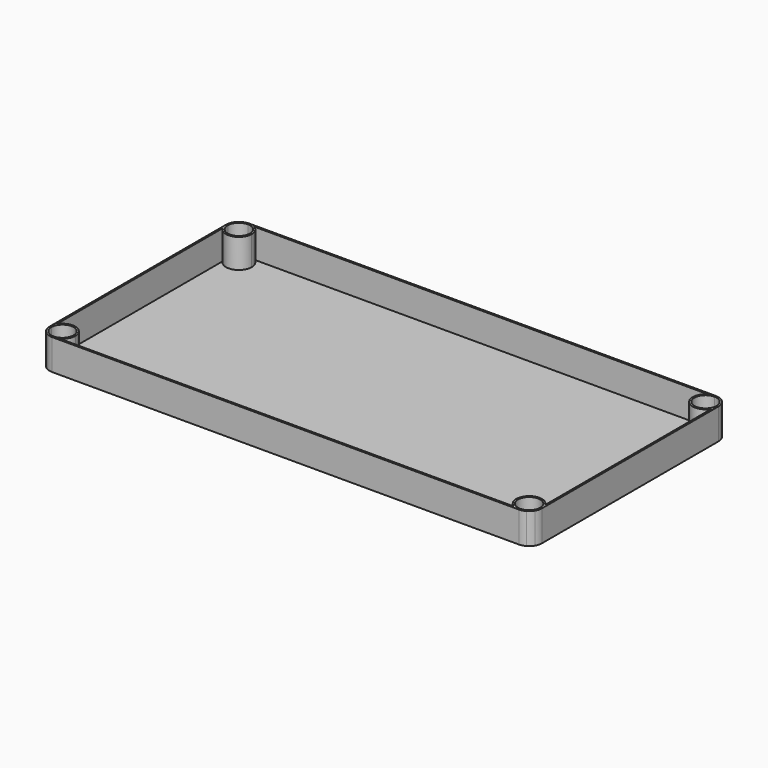
from build123d import *

# Parameters (mm, degrees)
F2_W     = 914.4
F2_H     = 457.2
F3_DEPTH = 57.15
F5_DEPTH = 53.975
F6_DEPTH = 57.15


# Not quite as in the source:
# - a length typed as a fraction of an inch, garbled in the dataset ("3 / 203.2 mm" for 3/8 in), is restored


with BuildPart() as f3:
    # F2 (on Top) → F3 (new body)
    with BuildSketch(Plane.XY):
        with Locations((457.2, 228.6)):
            Rectangle(F2_W, F2_H)
    extrude(amount=F3_DEPTH)

    # F4 (on face) → F5 (cut)
    with BuildSketch(Plane.XY.offset(57.15)):
        with BuildLine():
            ThreePointArc((47.625, 23.8125), (44.4270821412, 11.8930134592), (35.692262203, 3.175))
            Line((35.692262203, 3.175), (878.707737797, 3.175))
            ThreePointArc((878.707737797, 3.175), (873.749519773, 40.650480227), (911.225, 35.692262203))
            Line((911.225, 35.692262203), (911.225, 421.507737797))
            ThreePointArc((911.225, 421.507737797), (873.749519773, 416.549519773), (878.707737797, 454.025))
            Line((878.707737797, 454.025), (35.692262203, 454.025))
            ThreePointArc((35.692262203, 454.025), (44.4270821412, 445.3069865408), (47.625, 433.3875))
            ThreePointArc((47.625, 433.3875), (29.9608610621, 410.3824394154), (3.175, 421.507737797))
            Line((3.175, 421.507737797), (3.175, 35.692262203))
            ThreePointArc((3.175, 35.692262203), (29.9608610621, 46.8175605846), (47.625, 23.8125))
        make_face()
    extrude(amount=-F5_DEPTH, mode=Mode.SUBTRACT)

    # F4 (on face) → F6 (cut)
    with BuildSketch(Plane.XY.offset(57.15)):
        with BuildLine():
            Line((11.932737797, 3.175), (3.175, 3.175))
            Line((3.175, 3.175), (3.175, 11.932737797))
            ThreePointArc((3.175, 11.932737797), (0.8074394304, 17.6641388819), (0, 23.8124998841))
            Line((0, 23.8124998841), (0, 0))
            Line((0, 0), (23.8125, 0))
            ThreePointArc((23.8125, 0), (17.6641389379, 0.8074394154), (11.932737797, 3.175))
        make_face()
        with BuildLine():
            Line((3.175, 11.932737797), (3.175, 3.175))
            Line((3.175, 3.175), (11.932737797, 3.175))
            ThreePointArc((11.932737797, 3.175), (6.974519773, 6.974519773), (3.175, 11.932737797))
        make_face()
        with BuildLine():
            ThreePointArc((3.175, 23.8125001882), (9.2195837367, 9.2195838698), (23.8125, 3.175))
            ThreePointArc((23.8125, 3.175), (38.4054161967, 9.2195838033), (44.45, 23.8125))
            ThreePointArc((44.45, 23.8125), (23.8125000941, 44.45), (3.175, 23.8125001882))
        make_face()
        with BuildLine():
            ThreePointArc((23.8124998376, 454.025), (9.2195837458, 447.9804161393), (3.175, 433.3875))
            ThreePointArc((3.175, 433.3875), (23.8125, 412.75), (44.45, 433.3875))
            ThreePointArc((44.45, 433.3875), (38.4054161393, 447.9804162542), (23.8124998376, 454.025))
        make_face()
        with BuildLine():
            Line((3.175, 454.025), (3.175, 445.267262203))
            ThreePointArc((3.175, 445.267262203), (6.974519773, 450.225480227), (11.932737797, 454.025))
            Line((11.932737797, 454.025), (3.175, 454.025))
        make_face()
        with BuildLine():
            Line((0, 457.2), (0, 433.3875))
            ThreePointArc((0, 433.3875), (0.8074394154, 439.5358610621), (3.175, 445.267262203))
            Line((3.175, 445.267262203), (3.175, 454.025))
            Line((3.175, 454.025), (11.932737797, 454.025))
            ThreePointArc((11.932737797, 454.025), (17.6641390246, 456.3925606078), (23.8125001795, 457.2))
            Line((23.8125001795, 457.2), (0, 457.2))
        make_face()
        with BuildLine():
            ThreePointArc((902.467262203, 454.025), (907.425480227, 450.225480227), (911.225, 445.267262203))
            Line((911.225, 445.267262203), (911.225, 454.025))
            Line((911.225, 454.025), (902.467262203, 454.025))
        make_face()
        with BuildLine():
            ThreePointArc((911.225, 445.267262203), (913.5925605846, 439.5358610621), (914.4, 433.3875))
            Line((914.4, 433.3875), (914.4, 457.2))
            Line((914.4, 457.2), (890.5875, 457.2))
            ThreePointArc((890.5875, 457.2), (896.7358610621, 456.3925605846), (902.467262203, 454.025))
            Line((902.467262203, 454.025), (911.225, 454.025))
            Line((911.225, 454.025), (911.225, 445.267262203))
        make_face()
        with BuildLine():
            ThreePointArc((890.5875, 454.025), (875.9945838033, 418.7945838033), (911.225, 433.3875))
            ThreePointArc((911.225, 433.3875), (905.1804161967, 447.9804161967), (890.5875, 454.025))
        make_face()
        with BuildLine():
            ThreePointArc((911.225, 11.932737797), (907.425480227, 6.974519773), (902.467262203, 3.175))
            Line((902.467262203, 3.175), (911.225, 3.175))
            Line((911.225, 3.175), (911.225, 11.932737797))
        make_face()
        with BuildLine():
            ThreePointArc((902.467262203, 3.175), (896.7358610621, 0.8074394154), (890.5875, 0))
            Line((890.5875, 0), (914.4, 0))
            Line((914.4, 0), (914.4, 23.8125))
            ThreePointArc((914.4, 23.8125), (913.5925605846, 17.6641389379), (911.225, 11.932737797))
            Line((911.225, 11.932737797), (911.225, 3.175))
            Line((911.225, 3.175), (902.467262203, 3.175))
        make_face()
        with BuildLine():
            ThreePointArc((911.225, 23.8125), (875.9945838033, 38.4054161967), (890.5875, 3.175))
            ThreePointArc((890.5875, 3.175), (905.1804161967, 9.2195838033), (911.225, 23.8125))
        make_face()
    extrude(amount=-F6_DEPTH, mode=Mode.SUBTRACT)


solid = f3.part
